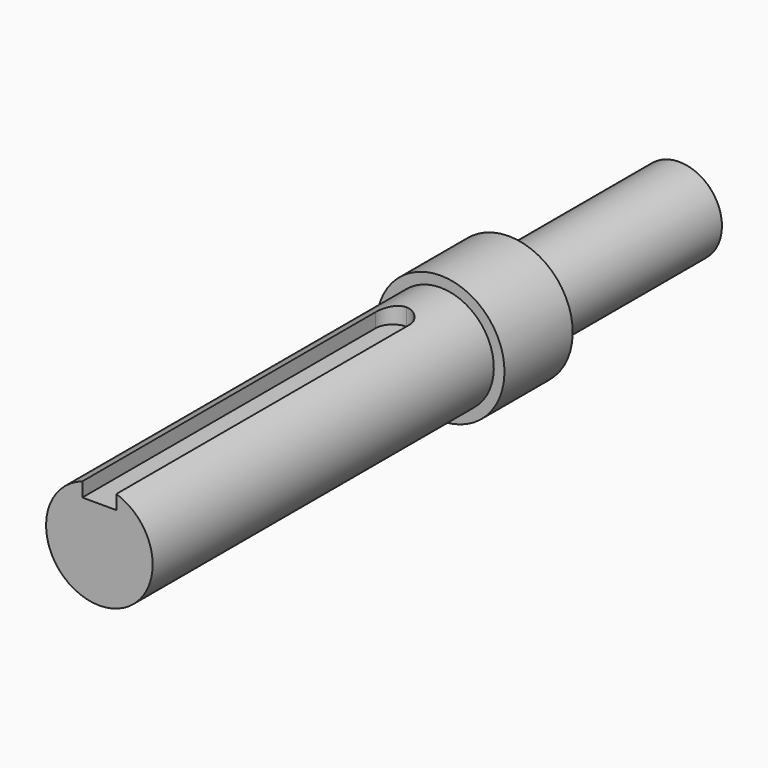
from build123d import *

# Parameters (mm, degrees)
F2_W     = 8
F2_H     = 4
F3_DEPTH = 90
F4_R     = 3.99999


# Not quite as in the source:
# - a fillet or chamfer is up to 0.001 mm smaller than in the source, because OpenCascade refuses the exact size


with BuildPart() as f1:
    # F0 (on Right) → F1 (revolve)
    with BuildSketch(Plane.YZ):
        Polygon((-110, 12.5), (-110, 0), (60, 0), (60, 10), (10, 10), (10, 15), (-10, 15), (-10, 12.5), align=None)
    revolve(axis=Axis((0, -25, 0), (0, -1, 0)))

    # F2 (on face) → F3 (cut)
    with BuildSketch(Plane.XZ.offset(110)):
        with Locations((0, 10.5)):
            Rectangle(F2_W, F2_H)
    extrude(amount=-F3_DEPTH, mode=Mode.SUBTRACT)

    # F4 (radius 4 in the source; OpenCascade refuses exactly that, so slightly less here)
    f4_edges = [f1.edges().sort_by_distance(p)[0] for p in [
        (-4, -20, 10.17136),
        (4, -20, 10.17136),
    ]]
    fillet(f4_edges, radius=F4_R)


solid = f1.part
